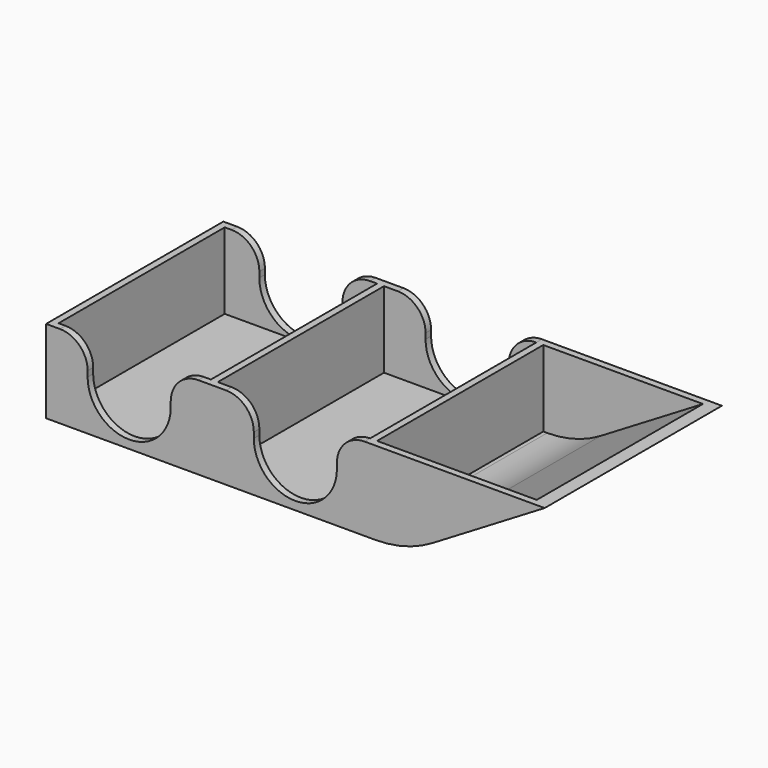
from build123d import *

# Parameters (mm, degrees)
F1_DEPTH = 101.6
F2_R     = 50.8
F3_T     = -3.175
F4_W     = 3.175
F4_H     = 95.25
F5_DEPTH = 34.925
F7_DEPTH = 101.601
F8_R     = 12.7


with BuildPart() as f1:
    # F0 (on Front) → F1 (new body)
    with BuildSketch(Plane.XZ):
        Polygon((0, 38.1), (0, 0), (165.1, 0), (228.6, 38.1), align=None)
    extrude(amount=F1_DEPTH)

    # F2
    f2_edges = [f1.edges().sort_by_distance(p)[0] for p in [
        (165.1, -50.8, 0),
    ]]
    fillet(f2_edges, radius=F2_R)

    # F3
    f3_openings = [f1.faces().sort_by_distance(p)[0] for p in [
        (114.3, -50.8, 38.1),
    ]]
    offset(amount=F3_T, openings=f3_openings)

    # F4 (on face) → F5 (join, through all)
    with BuildSketch(Plane.XY.offset(3.175)):
        with Locations((74.6125, -50.8)):
            Rectangle(F4_W, F4_H)
        with Locations((147.6375, -50.8)):
            Rectangle(F4_W, F4_H)
    extrude(amount=F5_DEPTH)

    # F6 (on face) → F7 (cut, through all)
    with BuildSketch(Plane.XZ.offset(101.6)):
        with BuildLine():
            Line((57.15, 38.1), (19.05, 38.1))
            Line((19.05, 38.1), (19.05, 22.86))
            ThreePointArc((19.05, 22.86), (38.1, 3.81), (57.15, 22.86))
            Line((57.15, 22.86), (57.15, 38.1))
        make_face()
        with BuildLine():
            Line((133.35, 38.1), (95.25, 38.1))
            Line((95.25, 38.1), (95.25, 22.86))
            ThreePointArc((95.25, 22.86), (114.3, 3.81), (133.35, 22.86))
            Line((133.35, 22.86), (133.35, 38.1))
        make_face()
    extrude(amount=-F7_DEPTH, mode=Mode.SUBTRACT)

    # F8
    f8_edges = [f1.edges().sort_by_distance(p)[0] for p in [
        (19.05, -100.0125, 38.1),
        (57.15, -100.0125, 38.1),
        (19.05, -1.5875, 38.1),
        (57.15, -1.5875, 38.1),
        (95.25, -100.0125, 38.1),
        (133.35, -100.0125, 38.1),
        (133.35, -1.5875, 38.1),
        (95.25, -1.5875, 38.1),
    ]]
    fillet(f8_edges, radius=F8_R)


solid = f1.part
